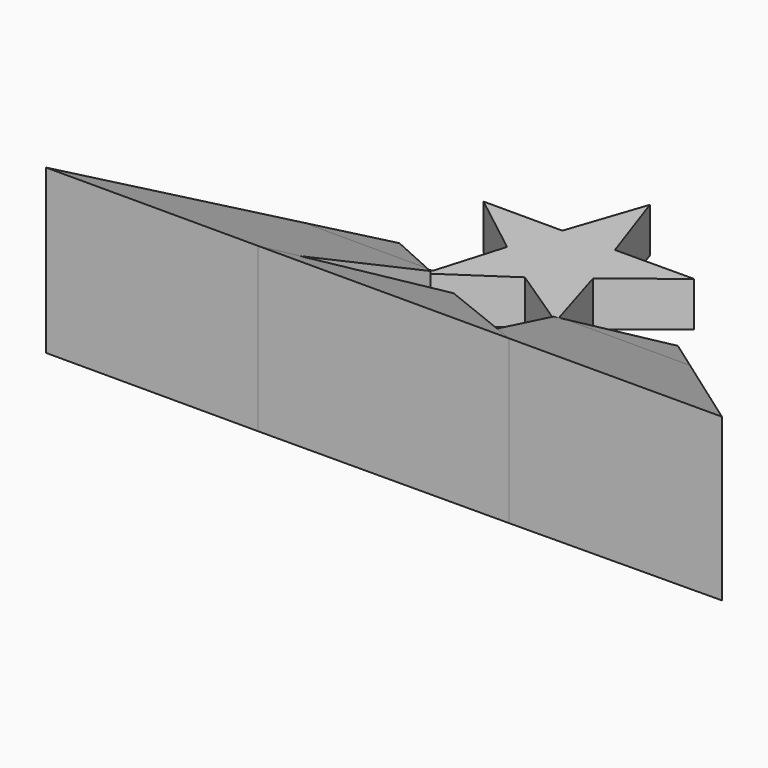
from build123d import *

# Parameters (mm, degrees)
F1_DEPTH      = 7
F2_DEPTH      = 7
F3_DEPTH      = 25
F4_DEPTH      = 25
F5_DEPTH      = 25
F6_DEPTH      = 25
F8_DEPTH      = 52.8462768922
F8_DEPTH_BACK = 52.8629522723


with BuildPart() as f1:
    # F0 (on Top) → F1 (new body)
    with BuildSketch(Plane.XY):
        Polygon((-21.854923692, 37.1773435624), (-22.2325250506, 36.8059538305), (-52.8452768922, 6.6967885941), (-19.641056972, 6.6967885941), (-15.9451588988, 9.3006277457), (-15.3760976448, 9.7015435566), (-9.7015127861, 28.0367903236), (-10.566638607, 28.6874495242), align=None)
    extrude(amount=F1_DEPTH)

    # F3#2 (add): a face of the model
    f3_2_faces = [f1.faces().sort_by_distance(p)[0] for p in [
        (-27.1983175925, 18.5191974615, 7),
    ]]
    extrude(f3_2_faces, amount=F3_DEPTH)

    # F0 (on Top) → F4, piece 2 (join)
    with BuildSketch(Plane.XY):
        Polygon((-21.854923692, 37.1773435624), (-22.2325250506, 36.8059538305), (-52.8452768922, 6.6967885941), (-19.641056972, 6.6967885941), (-15.9451588988, 9.3006277457), (-15.3760976448, 9.7015435566), (-9.7015127861, 28.0367903236), (-10.566638607, 28.6874495242), align=None)
    extrude(amount=-F4_DEPTH)


with BuildPart() as f1b:
    # F0 (on Top) → F1, piece 2 (new body)
    with BuildSketch(Plane.XY):
        Polygon((15.9488124875, 9.3834251701), (19.6581798972, 6.7988102444), (52.8619522723, 6.9712067974), (22.0932860403, 36.9210245738), (21.713761513, 37.2904487909), (10.4473401343, 28.7250548337), (9.6079722369, 28.0869181552), (15.3776773458, 9.7813810071), align=None)
    extrude(amount=F1_DEPTH)

    # F3 (add): a face of the model
    f3_faces = [f1b.faces().sort_by_distance(p)[0] for p in [
        (27.1539566234, 18.6602971152, 7),
    ]]
    extrude(f3_faces, amount=F3_DEPTH)

    # F0 (on Top) → F4 (join)
    with BuildSketch(Plane.XY):
        Polygon((15.9488124875, 9.3834251701), (19.6581798972, 6.7988102444), (52.8619522723, 6.9712067974), (22.0932860403, 36.9210245738), (21.713761513, 37.2904487909), (10.4473401343, 28.7250548337), (9.6079722369, 28.0869181552), (15.3776773458, 9.7813810071), align=None)
    extrude(amount=-F4_DEPTH)


with BuildPart() as f2:
    # F0 (on Top) → F2 (new body)
    with BuildSketch(Plane.XY):
        Polygon((-15.9451588988, 9.3006277457), (-19.641056972, 6.6967885941), (19.6581798972, 6.7988102444), (15.9488124875, 9.3834251701), (15.3776773458, 9.7813810071), (-0.0271789608, 20.5151846831), (-15.3760976448, 9.7015435566), align=None)
    extrude(amount=F2_DEPTH)

    # F0 (on Top) → F5 (join)
    with BuildSketch(Plane.XY):
        Polygon((-15.9451588988, 9.3006277457), (-19.641056972, 6.6967885941), (19.6581798972, 6.7988102444), (15.9488124875, 9.3834251701), (15.3776773458, 9.7813810071), (-0.0271789608, 20.5151846831), (-15.3760976448, 9.7015435566), align=None)
    extrude(amount=-F5_DEPTH)

    # F6 (add): a face of the model
    f6_faces = [f2.faces().sort_by_distance(p)[0] for p in [
        (-0.0033520119, 11.3369278406, 7),
    ]]
    extrude(f6_faces, amount=F6_DEPTH)


with BuildPart() as f2b:
    # F0 (on Top) → F2, piece 2 (new body)
    with BuildSketch(Plane.XY):
        Polygon((-9.9289040496, 28.8884764516), (-10.566638607, 28.6874495242), (-9.7015127861, 28.0367903236), (-0.0635392434, 34.5213427361), (0, 34.4790702877), (9.6079722369, 28.0869181552), (10.4473401343, 28.7250548337), (9.9289040496, 28.8884764516), (9.837764806, 28.9172053984), (6.641519679, 39.484072189), (16.3754133549, 47.1329648367), (4.0123272981, 47.0687747382), (-0.1273227543, 59.0910619484), (-4.204497207, 47.0474436879), (-16.5677499026, 47.0474436879), (-6.794274319, 39.4491925836), align=None)
    extrude(amount=F2_DEPTH)


with BuildPart() as f8_tool:
    # F7 (on Right) → F8 (new body, two sides)
    with BuildSketch(Plane.YZ) as f8_sk:
        Polygon((28.9172053984, 7), (37.2904487909, 3.5), (40.2094684541, 37.8902927041), (3.4889901212, 37.8902927041), (3.4889901212, 17.6289461917), align=None)
        Polygon((40.2094684541, -30.8902927041), (37.2904487909, 3.5), (28.9172053984, 0), (3.4889901212, -10.6289461917), (3.4889901212, -30.8902927041), align=None)
    extrude(amount=-F8_DEPTH)
    extrude(f8_sk.sketch, amount=F8_DEPTH_BACK)


with BuildPart() as f1_1:
    add(f1.part)

    # F8: cut by f8_tool
    add(f8_tool.part, mode=Mode.SUBTRACT)


with BuildPart() as f1b_1:
    add(f1b.part)

    # F8: cut by f8_tool
    add(f8_tool.part, mode=Mode.SUBTRACT)


with BuildPart() as f2_1:
    add(f2.part)

    # F8: cut by f8_tool
    add(f8_tool.part, mode=Mode.SUBTRACT)


solid = Compound([f2b.part, f1_1.part, f1b_1.part, f2_1.part])
